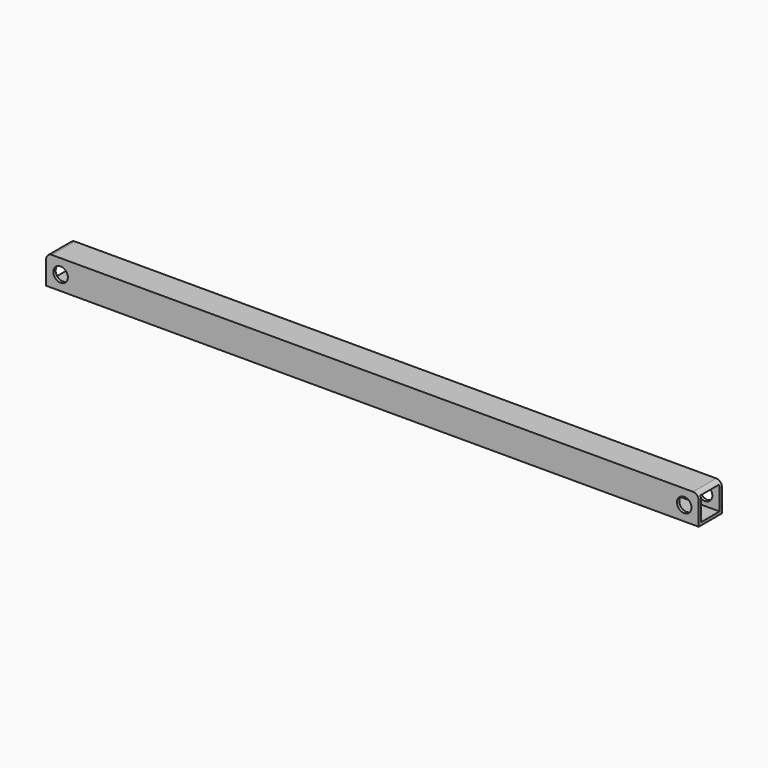
from build123d import *

# Parameters (mm, degrees)
F0_W        = 20
F0_H        = 20
F0_W_2      = 16
F0_H_2      = 16
F1_DEPTH    = 450
F2_R        = 5
F3_DEPTH    = 20.001
F4_R        = 5
F5_DEPTH    = 20.001
F6_T1_DEPTH = 40
F7_T1_DEPTH = 40


# Not quite as in the source:
# - a fillet or chamfer that OpenCascade refuses, or shapes differently, is made with other operations: its cross-section is extruded or revolved along the edge and cut away or added


with BuildPart() as f1:
    # F0 (on Right) → F1 (new body)
    with BuildSketch(Plane.YZ):
        with Locations((10, 10)):
            Rectangle(F0_W, F0_H)
        with Locations((10, 10)):
            Rectangle(F0_W_2, F0_H_2, mode=Mode.SUBTRACT)
    extrude(amount=F1_DEPTH)

    # F2 (on face) → F3 (cut, through all)
    with BuildSketch(Plane.XZ):
        with Locations((440, 10)):
            Circle(F2_R)
    extrude(amount=-F3_DEPTH, mode=Mode.SUBTRACT)

    # F4 (on face) → F5 (cut, through all)
    with BuildSketch(Plane.XZ):
        with Locations((10, 10)):
            Circle(F4_R)
    extrude(amount=-F5_DEPTH, mode=Mode.SUBTRACT)

    # F6: fillet of radius 4 on 1 edges, made by hand

    # F6_s2 → F6_t1 (cut)
    with BuildSketch(Plane.XZ.offset(-30)):
        with BuildLine():
            ThreePointArc((446, 20), (448.8284271247, 18.8284271247), (450, 16))
            Line((450, 16), (450, 20))
            Line((450, 20), (446, 20))
        make_face()
    extrude(amount=F6_T1_DEPTH, mode=Mode.SUBTRACT)

    # F7: fillet of radius 4 on 1 edges, made by hand

    # F7_s2 → F7_t1 (cut)
    with BuildSketch(Plane.XZ.offset(-30)):
        with BuildLine():
            ThreePointArc((0, 16), (1.1715728753, 18.8284271247), (4, 20))
            Line((4, 20), (0, 20))
            Line((0, 20), (0, 16))
        make_face()
    extrude(amount=F7_T1_DEPTH, mode=Mode.SUBTRACT)


solid = f1.part
